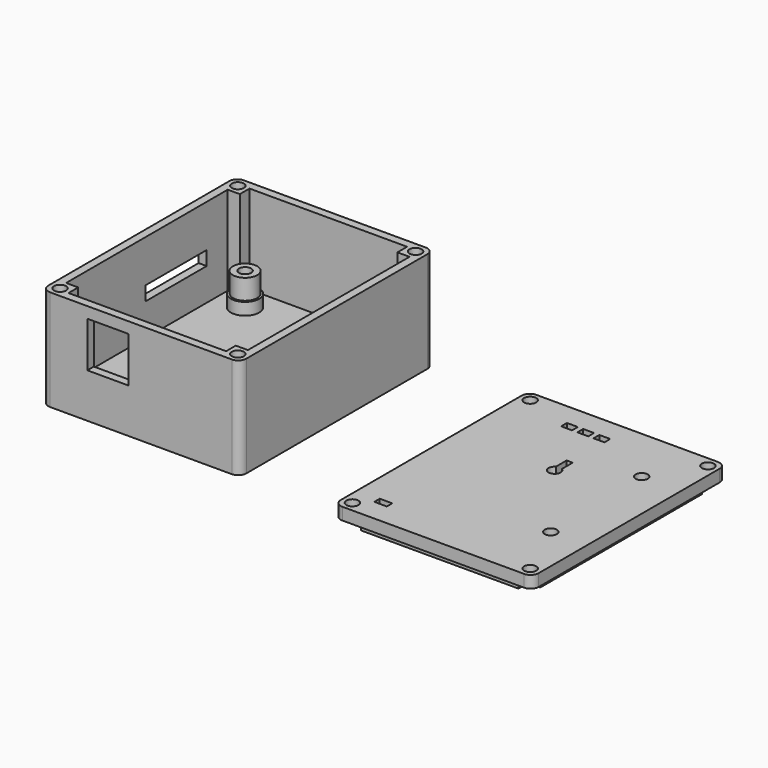
from build123d import *

# Parameters (mm, degrees)
F0_W      = 49
F0_H      = 60
F1_DEPTH  = 25
F2_W      = 39
F2_H      = 50
F3_DEPTH  = 22
F4_R      = 1.5
F5_DEPTH  = 8
F6_W      = 39
F6_H      = 3
F6_W_2    = 3
F6_H_2    = 50
F7_DEPTH  = 22
F8_R      = 3
F8_R_2    = 1.5
F9_DEPTH  = 8
F10_DEPTH = 11
F11_W     = 49
F11_H     = 60
F12_DEPTH = 3
F13_R     = 1.5
F14_DEPTH = 3
F15_W     = 10.2
F15_H     = 11.25
F16_DEPTH = 2
F17_W     = 19
F17_H     = 3.5
F18_DEPTH = 2
F19_R     = 3.5
F19_R_2   = 3
F20_DEPTH = 3
F21_R     = 1.5
F22_DEPTH = 2
F24_DEPTH = 3
F25_W     = 2.7
F25_H     = 1.8
F25_R     = 1.5
F25_W_2   = 3.11
F25_H_2   = 1.69
F26_DEPTH = 5
F28_DEPTH = 5
F29_R     = 2
F29_2_R   = 2
F30_W     = 39
F30_H     = 50
F30_W_2   = 2.7
F30_H_2   = 1.8
F30_R     = 1.5
F30_W_3   = 3.11
F30_H_3   = 1.69
F31_DEPTH = 2
F32_W     = 3
F32_H     = 50
F32_W_2   = 39
F32_H_2   = 3
F33_DEPTH = 2


# Not quite as in the source:
# - ends of sketch curves that miss each other by under 0.0002 mm in the source are joined
# - a feature names something its author has since deleted; it is built from what else it names


with BuildPart() as f1:
    # F0 (on Top) → F1 (new body)
    with BuildSketch(Plane.XY):
        with Locations((-42.2749249265, 37.3531144334)):
            Rectangle(F0_W, F0_H)
    extrude(amount=F1_DEPTH)

    # F2 (on face) → F3 (cut)
    with BuildSketch(Plane.XY.offset(25)):
        with Locations((-42.2749249265, 37.3531144334)):
            Rectangle(F2_W, F2_H)
    extrude(amount=-F3_DEPTH, mode=Mode.SUBTRACT)

    # F4 (on face) → F5 (cut)
    with BuildSketch(Plane.XY.offset(25)):
        with Locations((-20.2749249265, 64.8531144334)):
            Circle(F4_R)
        with Locations((-20.2749249265, 9.8531144334)):
            Circle(F4_R)
        with Locations((-64.2749249265, 9.8531144334)):
            Circle(F4_R)
        with Locations((-64.2749249265, 64.8531144334)):
            Circle(F4_R)
    extrude(amount=-F5_DEPTH, mode=Mode.SUBTRACT)

    # F6 (on face) → F7 (cut)
    with BuildSketch(Plane.XY.offset(25)):
        with Locations((-42.2749249265, 63.8531144334)):
            Rectangle(F6_W, F6_H)
        with Locations((-63.2749249265, 37.3531144334)):
            Rectangle(F6_W_2, F6_H_2)
        with Locations((-42.2749249265, 10.8531144334)):
            Rectangle(F6_W, F6_H)
        with Locations((-21.2749249265, 37.3531144334)):
            Rectangle(F6_W_2, F6_H_2)
    extrude(amount=-F7_DEPTH, mode=Mode.SUBTRACT)

    # F8 (on face) → F9 (join)
    with BuildSketch(Plane.XY.offset(3)):
        with Locations((-57.7749249265, 58.9731144334)):
            Circle(F8_R)
        with Locations((-57.7749249265, 58.9731144334)):
            Circle(F8_R_2, mode=Mode.SUBTRACT)
        with Locations((-25.3749249265, 15.3531144334)):
            Circle(F8_R)
        with Locations((-25.3749249265, 15.3531144334)):
            Circle(F8_R_2, mode=Mode.SUBTRACT)
    extrude(amount=F9_DEPTH)

    # F10 (cut): faces of the model
    f10_faces = [f1.faces().sort_by_distance(p)[0] for p in [
        (-25.3749249265, 15.3531144334, 3),
        (-57.7749249265, 58.9731144334, 3),
    ]]
    extrude(f10_faces, amount=-F10_DEPTH, mode=Mode.SUBTRACT)

    # F15 (on face) → F16 (cut)
    with BuildSketch(Plane.XZ.offset(-7.3531144334)):
        with Locations((-50.4249249265, 16.625)):
            Rectangle(F15_W, F15_H)
    extrude(amount=-F16_DEPTH, mode=Mode.SUBTRACT)

    # F17 (on face) → F18 (cut)
    with BuildSketch(Plane(origin=(-66.7749249265, 0, 0), x_dir=(0, -1, 0), z_dir=(-1, 0, 0))):
        with Locations((-46.3531144334, 12.75)):
            Rectangle(F17_W, F17_H)
    extrude(amount=-F18_DEPTH, mode=Mode.SUBTRACT)

    # F19 (on face) → F20 (join)
    with BuildSketch(Plane.XY.offset(3)):
        with Locations((-57.7749249265, 58.9731144334)):
            Circle(F19_R)
        with Locations((-57.7749249265, 58.9731144334)):
            Circle(F19_R_2, mode=Mode.SUBTRACT)
        with Locations((-25.3749249265, 15.3531144334)):
            Circle(F19_R)
        with Locations((-25.3749249265, 15.3531144334)):
            Circle(F19_R_2, mode=Mode.SUBTRACT)
    extrude(amount=F20_DEPTH)

    # F21 (on face) → F22 (cut)
    with BuildSketch(Plane(origin=(0, 0, 0), x_dir=(1, 0, 0), z_dir=(0, 0, -1))):
        Polygon((-54.782162725, -59.1813796625), (-56.0981808467, -56.485438954), (-59.0909430481, -56.277173725), (-60.7676871279, -58.7648492044), (-59.4516690063, -61.4607899128), (-56.4589068048, -61.6690551419), align=None)
        with Locations((-57.7749249265, -58.9731144334)):
            Circle(F21_R, mode=Mode.SUBTRACT)
        Polygon((-22.3787499739, -15.5045596509), (-23.7456820446, -12.8340734191), (-26.7418569971, -12.6826282016), (-28.371099879, -15.201669216), (-27.0041678083, -17.8721554478), (-24.0079928558, -18.0236006652), align=None)
        with Locations((-25.3749249265, -15.3531144334)):
            Circle(F21_R, mode=Mode.SUBTRACT)
    extrude(amount=-F22_DEPTH, mode=Mode.SUBTRACT)

    # F23 (on face) → F24 (cut)
    with BuildSketch(Plane.XY.offset(3)):
        with BuildLine():
            Line((-37.7749249265, 34.3531144334), (-33.7749249265, 34.3531144334))
            ThreePointArc((-33.7749249265, 34.3531144334), (-40.6033520512, 37.1815415582), (-37.7749249265, 30.3531144334))
            Line((-37.7749249265, 30.3531144334), (-37.7749249265, 34.3531144334))
        make_face()
        with BuildLine():
            ThreePointArc((-37.7749249265, 30.3531144334), (-34.9464978017, 31.5246873087), (-33.7749249265, 34.3531144334))
            Line((-33.7749249265, 34.3531144334), (-37.7749249265, 34.3531144334))
            Line((-37.7749249265, 34.3531144334), (-37.7749249265, 30.3531144334))
        make_face()
    extrude(amount=-F24_DEPTH, mode=Mode.SUBTRACT)

    # F29
    f29_edges = [f1.edges().sort_by_distance(p)[0] for p in [
        (-17.774925, 67.353114, 12.5),
        (-17.774925, 7.353114, 12.5),
        (-66.774925, 7.353114, 12.5),
        (-66.774925, 67.353114, 12.5),
    ]]
    fillet(f29_edges, radius=F29_R)


with BuildPart() as f12:
    # F11 (on Top) → F12 (new body)
    with BuildSketch(Plane.XY):
        with Locations((31.5337867644, 35.5543226007)):
            Rectangle(F11_W, F11_H)
    extrude(amount=F12_DEPTH)

    # F13 (on face) → F14 (cut)
    with BuildSketch(Plane.XY.offset(3)):
        with Locations((9.5337867644, 63.0543226007)):
            Circle(F13_R)
        with Locations((53.5337867644, 63.0543226007)):
            Circle(F13_R)
        with Locations((53.5337867644, 8.0543226007)):
            Circle(F13_R)
        with Locations((9.5337867644, 8.0543226007)):
            Circle(F13_R)
    extrude(amount=-F14_DEPTH, mode=Mode.SUBTRACT)

    # F25 (on face) → F26 (cut)
    with BuildSketch(Plane.XY.offset(3)):
        with Locations((22.3837867644, 59.1543226007)):
            Rectangle(F25_W, F25_H)
        with Locations((26.3937867644, 59.1543226007)):
            Rectangle(F25_W, F25_H)
        with Locations((30.3937867644, 59.1543226007)):
            Rectangle(F25_W, F25_H)
        with Locations((46.3237867644, 51.5543226007)):
            Circle(F25_R)
        with Locations((47.0837867644, 22.4943226007)):
            Circle(F25_R)
        with Locations((14.1287867644, 11.8593226007)):
            Rectangle(F25_W_2, F25_H_2)
    extrude(amount=-F26_DEPTH, mode=Mode.SUBTRACT)

    # F27 (on face) → F28 (cut)
    with BuildSketch(Plane.XY.offset(3)):
        with BuildLine():
            ThreePointArc((30.7837702638, 44.4063511796), (31.5337867644, 44.6073226007), (32.2838032649, 44.4063511796))
            Line((32.2838032649, 44.4063511796), (32.2837867644, 47.7683226007))
            Line((32.2837867644, 47.7683226007), (30.7837867644, 47.7683226007))
            Line((30.7837867644, 47.7683226007), (30.7837702638, 44.4063511796))
        make_face()
        with BuildLine():
            ThreePointArc((30.7837702638, 44.4063511796), (30.7837950147, 41.8082797317), (33.0337867644, 43.1073226007))
            ThreePointArc((33.0337867644, 43.1073226007), (32.8328296333, 43.8573143503), (32.2838032649, 44.4063511796))
            ThreePointArc((32.2838032649, 44.4063511796), (31.5337867644, 44.6073226007), (30.7837702638, 44.4063511796))
        make_face()
    extrude(amount=-F28_DEPTH, mode=Mode.SUBTRACT)

    # F29#2
    f29_2_edges = [f12.edges().sort_by_distance(p)[0] for p in [
        (56.033787, 65.554323, 1.5),
        (56.033787, 5.554323, 1.5),
        (7.033787, 65.554323, 1.5),
        (7.033787, 5.554323, 1.5),
    ]]
    fillet(f29_2_edges, radius=F29_2_R)

    # F30 (on face) → F31 (join)
    with BuildSketch(Plane(origin=(0, 0, 0), x_dir=(1, 0, 0), z_dir=(0, 0, -1))):
        with Locations((31.5337867644, -35.5543226007)):
            Rectangle(F30_W, F30_H)
        with Locations((22.3837867644, -59.1543226007)):
            Rectangle(F30_W_2, F30_H_2, mode=Mode.SUBTRACT)
        with Locations((26.3937867644, -59.1543226007)):
            Rectangle(F30_W_2, F30_H_2, mode=Mode.SUBTRACT)
        with Locations((30.3937867644, -59.1543226007)):
            Rectangle(F30_W_2, F30_H_2, mode=Mode.SUBTRACT)
        with Locations((46.3237867644, -51.5543226007)):
            Circle(F30_R, mode=Mode.SUBTRACT)
        with BuildLine():
            ThreePointArc((30.7837702638, -44.4063511796), (31.5337867644, -41.6073226007), (32.2838032649, -44.4063511796))
            Line((32.2838032649, -44.4063511796), (32.2837867644, -47.7683226007))
            Line((32.2837867644, -47.7683226007), (30.7837867644, -47.7683226007))
            Line((30.7837867644, -47.7683226007), (30.7837702638, -44.4063511796))
        make_face(mode=Mode.SUBTRACT)
        with Locations((14.1287867644, -11.8593226007)):
            Rectangle(F30_W_3, F30_H_3, mode=Mode.SUBTRACT)
        with Locations((47.0837867644, -22.4943226007)):
            Circle(F30_R, mode=Mode.SUBTRACT)
    extrude(amount=F31_DEPTH)

    # F32 (on face) → F33 (join)
    with BuildSketch(Plane(origin=(0, 0, 0), x_dir=(1, 0, 0), z_dir=(0, 0, -1))):
        with Locations((10.5337867644, -35.5543226007)):
            Rectangle(F32_W, F32_H)
        with Locations((31.5337867644, -9.0543226007)):
            Rectangle(F32_W_2, F32_H_2)
        with Locations((52.5337867644, -35.5543226007)):
            Rectangle(F32_W, F32_H)
        with Locations((31.5337867644, -62.0543226007)):
            Rectangle(F32_W_2, F32_H_2)
    extrude(amount=F33_DEPTH)


solid = Compound([f1.part, f12.part])
